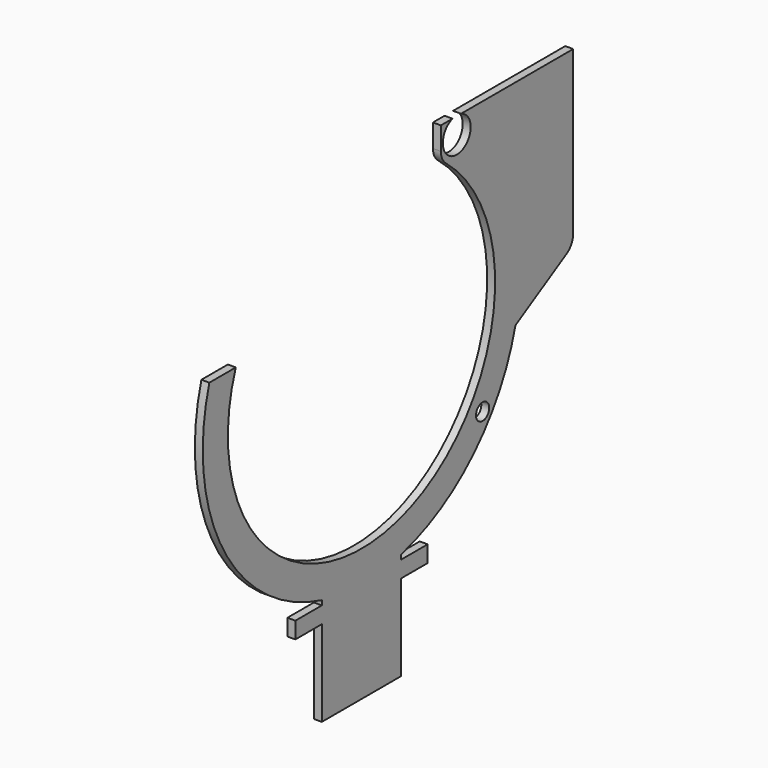
from build123d import *

# Parameters (mm, degrees)
F1_DEPTH     = 34
F2_R         = 5
F3_T         = -2.4
F5_DEPTH     = 31.6
F6_R         = 2.5
F7_DEPTH     = 34.001
F8_R         = 5
F9_T         = 2.4
F9_T3_DEPTH  = 10.7666522226
F9_T5_DEPTH  = 36.6379168457
F9_T7_DEPTH  = 39.0950180144
F9_T9_DEPTH  = 53.9897706946
F9_T11_DEPTH = 38.5655287546
F9_T13_DEPTH = 38.5655287546
F9_T15_DEPTH = 34
F9_T17_DEPTH = 38.8
F9_T20_ANGLE = 72.0602715047
F9_T22_ANGLE = 0.4928779222
F9_T24_ANGLE = 94.6188464687
F9_T26_ANGLE = 72.0602715047
F9_T28_ANGLE = 0.4928779222
F9_T30_ANGLE = 94.6188464687
F9_T32_ANGLE = 60.000000001
F9_T34_ANGLE = 60.000000001
F11_R        = 2.5
F12_DEPTH    = 4
F13_R        = 5
F13_R_2      = 2.5
F14_DEPTH    = 31.6
F15_W        = 10
F15_H        = 5
F16_DEPTH    = 34
F17_R        = 2.1082
F18_DEPTH    = 95.001
F19_W        = 187.0749369264
F19_H        = 174.4705922902
F20_DEPTH    = 31.601
F21_R        = 5.25
F22_DEPTH    = 2.401


# Not quite as in the source:
# - a shell that OpenCascade refuses in one call is made with other operations: the cavity is built on its own and cut out


with BuildPart() as f1:
    # F0 (on Right) → F1 (new body)
    with BuildSketch(Plane.YZ):
        with BuildLine():
            Line((28.1775091127, -64.6757430287), (50, -52.0765220406))
            Line((50, -52.0765220406), (50, 0))
            Line((50, 0), (0, 0))
            Line((0, 0), (0, -9.3767308061))
            ThreePointArc((0, -9.3767308061), (-15.3280037593, -98.3216569078), (-77.5220977637, -32.9149122293))
            Line((-77.5220977637, -32.9149122293), (-87.5160827584, -32.9149122293))
            ThreePointArc((-87.5160827584, -32.9149122293), (-82.2268855449, -79.5356128475), (-45, -108.0947501931))
            Line((-45, -108.0947501931), (-45, -140.5))
            Line((-45, -140.5), (-15, -140.5))
            Line((-15, -140.5), (-15, -108.0947501931))
            ThreePointArc((-15, -108.0947501931), (12.5445590619, -92.3079247214), (28.1775091127, -64.6757430287))
        make_face()
    extrude(amount=F1_DEPTH)

    # F2
    f2_edges = [f1.edges().sort_by_distance(p)[0] for p in [
        (17, 50, -52.076522),
        (17, 0, -9.376731),
    ]]
    fillet(f2_edges, radius=F2_R)

    # F3
    f3_openings = [f1.faces().sort_by_distance(p)[0] for p in [
        (17, 25, 0),
        (17, -16.449744, -98.64813),
        (17, 0.485259, -9.076135),
        (17, 0, -3.463693),
        (17, -82.51909, -32.914912),
        (17, -30, -140.5),
    ]]
    offset(amount=F3_T, openings=f3_openings, kind=Kind.INTERSECTION)

    # F4 (on face) → F5 (join, through all)
    with BuildSketch(Plane.YZ.offset(34)):
        with BuildLine():
            Line((-17.9050913084, -99.0302272455), (-17.9050913084, -108.768300841))
            ThreePointArc((-17.9050913084, -108.768300841), (12.6426107824, -92.2090955323), (28.8888176814, -61.493787543))
            Line((28.8888176814, -61.493787543), (17.0581943263, -68.3242011218))
            ThreePointArc((17.0581943263, -68.3242011218), (3.323976492, -87.9442036517), (-17.9050913084, -99.0302272455))
        make_face()
    extrude(amount=-F5_DEPTH)

    # F6 (on face) → F7 (cut, through all)
    with BuildSketch(Plane(origin=(0, 0, 0), x_dir=(0, -1, 0), z_dir=(-1, 0, 0))):
        with Locations((-6, -5)):
            Circle(F6_R)
        with Locations((-15.772, -82.60931)):
            Circle(F6_R)
    extrude(amount=-F7_DEPTH, mode=Mode.SUBTRACT)

    # F8
    f8_edges = [f1.edges().sort_by_distance(p)[0] for p in [
        (17, -17.905091, -99.030227),
    ]]
    fillet(f8_edges, radius=F8_R)

    # F9: shell of thickness 2.4, made by hand


with BuildPart() as f9_core1:
    # F9_t2: copy of F1
    add(f1.part)

    # the walls: a layer under each face that stays
    f9_faces = [f9_core1.faces().sort_by_distance(p)[0] for p in [
        (31.5714285714, 9.4533353128, -81.5227589639),
        (31.6, -26.6376443104, -122.5691520382),
        (17, -16.9486299393, -99.860595178),
        (28.3333333333, -85.8504185926, -32.9149122293),
        (2.4, -26.6376443104, -122.5691520382),
        (34, -20, -117.0833333333),
        (32.8, 0.4852593781, -9.0761346936),
        (31.6, 23.8, -34.1621005609),
        (0, -20, -117.0833333333),
        (17, 31.6790971631, -59.8828189331),
        (1.2, 0.4852593781, -9.0761346936),
        (2.4, 23.8, -34.1621005609),
        (17, -17.9050913084, -105.7849747297),
        (17, -17.6524314389, -108.7157351195),
        (17, -17.4, -124.5810415771),
        (31.5714285714, -42.8571428571, -140.5),
        (17, -42.6, -123.3524909928),
        (17, -79.8554185962, -78.8478289755),
        (17, -82.2268855449, -79.5356128475),
        (17, 37.8387545563, -59.0978203711),
        (17, 49.3301270189, -51.6897706946),
        (17, 50, -24.5948853473),
        (17, -15, -124.2973750966),
        (32.8666666667, 48.3333333333, 0),
        (32.8, 0, -3.4636934457),
        (17, -45, -124.2973750966),
        (17, 18.272, -82.60931),
        (32.8, 8.5, -5),
        (17, 47.6, -24.5948853473),
        (17, 47.2516660498, -50.4897706946),
        (1.2, 0, -3.4636934457),
        (1.2, 8.5, -5),
    ]]
    thicken(f9_faces, amount=-F9_T, mode=Mode.SUBTRACT)

    # F9_s4 → F9_t3 (cut)
    with BuildSketch(Plane.XY.offset(-111.168300841)):
        Polygon((31.576, -17.9290913084), (34, -17.9050913084), (34, -15.5050913084), (31.6, -15.5050913084), align=None)
        Polygon((2.424, -17.9290913084), (0, -17.9050913084), (0, -15.5050913084), (2.4, -15.5050913084), align=None)
    extrude(amount=F9_T3_DEPTH, mode=Mode.SUBTRACT)

    # F9_s6 → F9_t5 (cut)
    with BuildSketch(Plane.XY.offset(-142.9)):
        Polygon((31.576, -17.424), (34, -17.4), (34, -15), (31.6, -15), align=None)
        Polygon((2.424, -17.424), (0, -17.4), (0, -15), (2.4, -15), align=None)
    extrude(amount=F9_T5_DEPTH, mode=Mode.SUBTRACT)

    # F9_s8 → F9_t7 (cut)
    with BuildSketch(Plane.XY.offset(-142.9)):
        Polygon((31.576, -42.576), (34, -42.6), (34, -45), (31.6, -45), align=None)
        Polygon((2.424, -42.576), (0, -42.6), (0, -45), (2.4, -45), align=None)
    extrude(amount=F9_T7_DEPTH, mode=Mode.SUBTRACT)

    # F9_s10 → F9_t9 (cut)
    with BuildSketch(Plane.XY.offset(-51.5897706946)):
        Polygon((31.576, 47.576), (34, 47.6), (34, 50), (31.6, 50), align=None)
        Polygon((2.424, 47.576), (0, 47.6), (0, 50), (2.4, 50), align=None)
    extrude(amount=F9_T9_DEPTH, mode=Mode.SUBTRACT)

    # F9_s12 → F9_t11 (cut)
    with BuildSketch(Plane(origin=(0, 14.5286654552, 8.3881289115), x_dir=(1, 0, 0), z_dir=(0, -0.8660254038, -0.5))):
        Polygon((31.576, -67.6755910279), (34, -67.6995910279), (34, -70.0995910279), (31.6, -70.0995910279), align=None)
    extrude(amount=F9_T11_DEPTH, mode=Mode.SUBTRACT)

    # F9_s14 → F9_t13 (cut)
    with BuildSketch(Plane(origin=(0, -18.8700621567, -10.8946354658), x_dir=(1, 0, 0), z_dir=(0, 0.8660254038, 0.5))):
        Polygon((2.424, 67.6755910279), (2.4, 70.0995910279), (0, 70.0995910279), (0, 67.6995910279), align=None)
    extrude(amount=F9_T13_DEPTH, mode=Mode.SUBTRACT)

    # F9_s16 → F9_t15 (cut)
    with BuildSketch(Plane.YZ):
        Polygon((-17.41896, -108.6855479875), (-17.904, -106.3155998281), (-15, -105.6918510958), (-15, -108.6620831543), align=None)
    extrude(amount=F9_T15_DEPTH, mode=Mode.SUBTRACT)

    # F9_s18 → F9_t17 (cut)
    with BuildSketch(Plane.YZ.offset(-2.4)):
        Polygon((-45.03, -108.1179880932), (-44.4, -105.7709601854), (-42.6, -106.2357181869), (-42.6, -108.0947501931), align=None)
    extrude(amount=F9_T17_DEPTH, mode=Mode.SUBTRACT)

    # F9_s19 → F9_t20 (revolve, cut)
    with BuildSketch(Plane(origin=(0, -41.8058245271, -13.5349325593), x_dir=(1, 0, 0), z_dir=(0, 0.9513810562, 0.3080163728))):
        Polygon((31.576, 88.8045616247), (34, 88.8285616247), (34, 91.2285616247), (31.6, 91.2285616247), align=None)
    revolve(axis=Axis((31.6, -12.9050913084, -102.8016486184), (1, 0, 0)), revolution_arc=F9_T20_ANGLE, mode=Mode.SUBTRACT)

    # F9_s21 → F9_t22 (revolve, cut)
    with BuildSketch(Plane(origin=(0, -38.6531269844, -7.9550716089), x_dir=(1, 0, 0), z_dir=(0, -0.9794716807, -0.2015818115))):
        Polygon((31.576, -102.9501296884), (34, -102.9261296884), (34, -100.5261296884), (31.6, -100.5261296884), align=None)
    revolve(axis=Axis((31.6, -30, -50), (1, 0, 0)), revolution_arc=F9_T22_ANGLE, mode=Mode.SUBTRACT)

    # F9_s23 → F9_t24 (revolve, cut)
    with BuildSketch(Plane(origin=(0, -17.8918491238, 4.0109842757), x_dir=(1, 0, 0), z_dir=(0, 0.9757809372, -0.21875))):
        Polygon((31.576, 112.9275468625), (34, 112.9515468625), (34, 115.3515468625), (31.6, 115.3515468625), align=None)
    revolve(axis=Axis((31.6, -30, -50), (-1, 0, 0)), revolution_arc=F9_T24_ANGLE, mode=Mode.SUBTRACT)

    # F9_s25 → F9_t26 (revolve, cut)
    with BuildSketch(Plane(origin=(0, -41.8058245271, -13.5349325593), x_dir=(1, 0, 0), z_dir=(0, 0.9513810562, 0.3080163728))):
        Polygon((2.424, 88.8045616247), (2.4, 91.2285616247), (0, 91.2285616247), (0, 88.8285616247), align=None)
    revolve(axis=Axis((2.4, -12.9050913084, -102.8016486184), (1, 0, 0)), revolution_arc=F9_T26_ANGLE, mode=Mode.SUBTRACT)

    # F9_s27 → F9_t28 (revolve, cut)
    with BuildSketch(Plane(origin=(0, -38.6531269844, -7.9550716089), x_dir=(1, 0, 0), z_dir=(0, -0.9794716807, -0.2015818115))):
        Polygon((2.424, -102.9501296884), (0, -102.9261296884), (0, -100.5261296884), (2.4, -100.5261296884), align=None)
    revolve(axis=Axis((2.4, -30, -50), (1, 0, 0)), revolution_arc=F9_T28_ANGLE, mode=Mode.SUBTRACT)

    # F9_s29 → F9_t30 (revolve, cut)
    with BuildSketch(Plane(origin=(0, -17.8918491238, 4.0109842757), x_dir=(1, 0, 0), z_dir=(0, 0.9757809372, -0.21875))):
        Polygon((2.424, 112.9275468625), (0, 112.9515468625), (0, 115.3515468625), (2.4, 115.3515468625), align=None)
    revolve(axis=Axis((2.4, -30, -50), (-1, 0, 0)), revolution_arc=F9_T30_ANGLE, mode=Mode.SUBTRACT)

    # F9_s31 → F9_t32 (revolve, cut)
    with BuildSketch(Plane(origin=(0, 12.4502044861, 7.1881289115), x_dir=(1, 0, 0), z_dir=(0, -0.8660254038, -0.5))):
        Polygon((31.576, -67.6755910279), (34, -67.6995910279), (34, -70.0995910279), (31.6, -70.0995910279), align=None)
    revolve(axis=Axis((31.6, 45, -49.1897706946), (1, 0, 0)), revolution_arc=F9_T32_ANGLE, mode=Mode.SUBTRACT)

    # F9_s33 → F9_t34 (revolve, cut)
    with BuildSketch(Plane(origin=(0, 12.4502044861, 7.1881289115), x_dir=(1, 0, 0), z_dir=(0, -0.8660254038, -0.5))):
        Polygon((2.424, -67.6755910279), (0, -67.6995910279), (0, -70.0995910279), (2.4, -70.0995910279), align=None)
    revolve(axis=Axis((2.4, 45, -49.1897706946), (1, 0, 0)), revolution_arc=F9_T34_ANGLE, mode=Mode.SUBTRACT)


with BuildPart() as f1_1:
    add(f1.part)

    # what is left inside the walls is the cavity
    f9_cavity = [f9_core1.part.solids().sort_by_distance(p)[0] for p in [
        (21.866667, 25.090457, -73.709958),
        (21.866667, 2.64665, -100.312194),
    ]]
    add(f9_cavity, mode=Mode.SUBTRACT)

    # F11 (on offset) → F12 (join)
    with BuildSketch(Plane.YZ.offset(9.4)):
        with BuildLine():
            Line((47.6, -49.1897706946), (47.6, 0))
            Line((47.6, 0), (0, 0))
            Line((0, 0), (0, -6.9273868914))
            ThreePointArc((0, -6.9273868914), (0.4852593781, -9.0761346936), (1.8468468468, -10.8078024868))
            ThreePointArc((1.8468468468, -10.8078024868), (18.82146463, -37.0881995298), (17.0581943263, -68.3242011218))
            Line((17.0581943263, -68.3242011218), (46.3, -51.4414367444))
            ThreePointArc((46.3, -51.4414367444), (47.2516660498, -50.4897706946), (47.6, -49.1897706946))
        make_face()
        with Locations((6, -5)):
            Circle(F11_R, mode=Mode.SUBTRACT)
    extrude(amount=F12_DEPTH)

    # F13 (on face) → F14 (join, through all)
    with BuildSketch(Plane(origin=(0, 0, 0), x_dir=(0, -1, 0), z_dir=(-1, 0, 0))):
        with Locations((-6, -5)):
            Circle(F13_R)
        with Locations((-6, -5)):
            Circle(F13_R_2, mode=Mode.SUBTRACT)
    extrude(amount=-F14_DEPTH)

    # F15 (on face) → F16 (join, through all)
    with BuildSketch(Plane(origin=(0, 0, 0), x_dir=(0, -1, 0), z_dir=(-1, 0, 0))):
        with Locations((50, -111.9852015376)):
            Rectangle(F15_W, F15_H)
        with Locations((10, -111.9852015376)):
            Rectangle(F15_W, F15_H)
    extrude(amount=-F16_DEPTH)

    # F17 (on face) → F18 (cut, through all)
    with BuildSketch(Plane.XZ.offset(45)):
        with Locations((17, -127.4926007688)):
            Circle(F17_R)
    extrude(amount=-F18_DEPTH, mode=Mode.SUBTRACT)

    # F19 (on face) → F20 (cut, through all)
    with BuildSketch(Plane.YZ.offset(2.4)):
        with Locations((-24.4173072278, -67.2780927271)):
            Rectangle(F19_W, F19_H)
    extrude(amount=F20_DEPTH, mode=Mode.SUBTRACT)

    # F21 (on face) → F22 (cut, through all)
    with BuildSketch(Plane.YZ.offset(2.4)):
        with Locations((6, -5)):
            Circle(F21_R)
    extrude(amount=-F22_DEPTH, mode=Mode.SUBTRACT)


solid = f1_1.part
